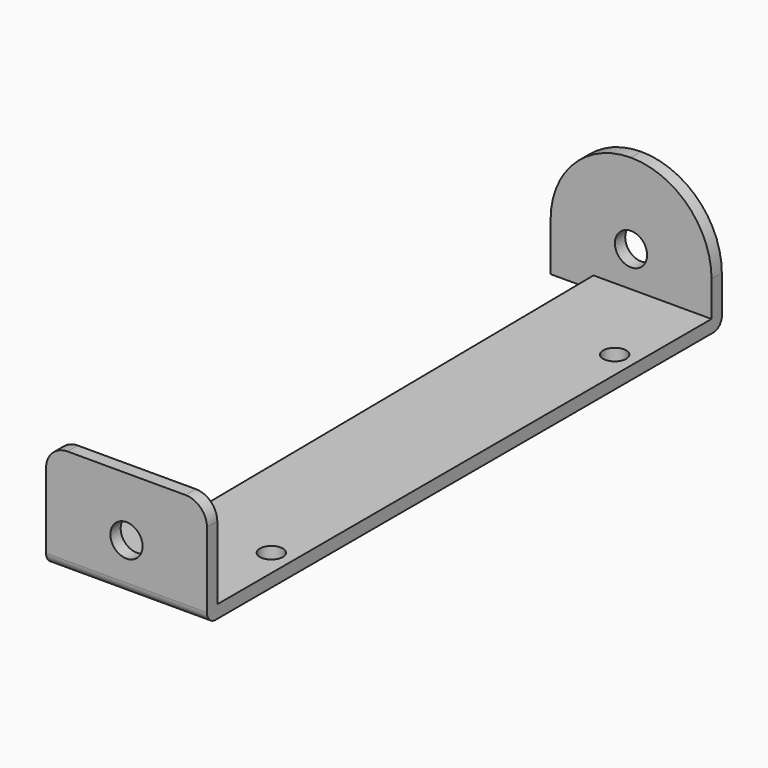
from build123d import *

# Parameters (mm, degrees)
F0_R        = 1.075
F3_DEPTH    = 1.2
F2_W        = 15
F2_H        = 1.2
F4_DEPTH    = 10
F1_W        = 15
F1_H        = 1.2
F5_DEPTH    = 12
F6_T1_DEPTH = 38.762491
F7_R        = 2
F8_R        = 1
F10_D       = 3


# Not quite as in the source:
# - a fillet or chamfer that OpenCascade refuses, or shapes differently, is made with other operations: its cross-section is extruded or revolved along the edge and cut away or added


with BuildPart() as f3:
    # F0 (on Top) → F3 (new body)
    with BuildSketch(Plane.XY):
        Polygon((-15, 0), (0, 0), (0, 60), (-15, 60), (-15, 58.8), (-11, 58.8), (-10.4650629229, 8.8028616587), (-15, 7), align=None)
        with Locations((-2, 10)):
            Circle(F0_R, mode=Mode.SUBTRACT)
        with Locations((-2, 50)):
            Circle(F0_R, mode=Mode.SUBTRACT)
    extrude(amount=F3_DEPTH)

    # F2 (on face) → F4 (join)
    with BuildSketch(Plane.XY):
        with Locations((-7.5, 0.6)):
            Rectangle(F2_W, F2_H)
    extrude(amount=F4_DEPTH)

    # F1 (on face) → F5 (join)
    with BuildSketch(Plane.XY):
        with Locations((-7.5, 59.3886146865)):
            Rectangle(F1_W, F1_H)
    extrude(amount=F5_DEPTH)

    # F6: fillet of radius 7.5124982 on 2 edges, made by hand

    # F6_s2 → F6_t1 (cut)
    with BuildSketch(Plane.XZ.offset(-78.7698601865)):
        with BuildLine():
            ThreePointArc((0, 4.4875018), (-2.2003597791, 9.7996402209), (-7.5124982, 12))
            Line((-7.5124982, 12), (0, 12))
            Line((0, 12), (0, 4.4875018))
        make_face()
        with BuildLine():
            ThreePointArc((-15, 4.4875018), (-12.7996402209, 9.7996402209), (-7.4875018, 12))
            Line((-7.4875018, 12), (-15, 12))
            Line((-15, 12), (-15, 4.4875018))
        make_face()
    extrude(amount=F6_T1_DEPTH, mode=Mode.SUBTRACT)

    # F7
    f7_edges = [f3.edges().sort_by_distance(p)[0] for p in [
        (0, 0.6, 10),
        (-15, 0.6, 10),
    ]]
    fillet(f7_edges, radius=F7_R)

    # F8
    f8_edges = [f3.edges().sort_by_distance(p)[0] for p in [
        (-7.5, 0, 0),
        (-7.5, 60, 0),
    ]]
    fillet(f8_edges, radius=F8_R)

    # F10 (through all)
    with Locations(Plane.XZ):
        with Locations((-7.506201975, 4.490504507)):
            Hole(F10_D / 2)


solid = f3.part
